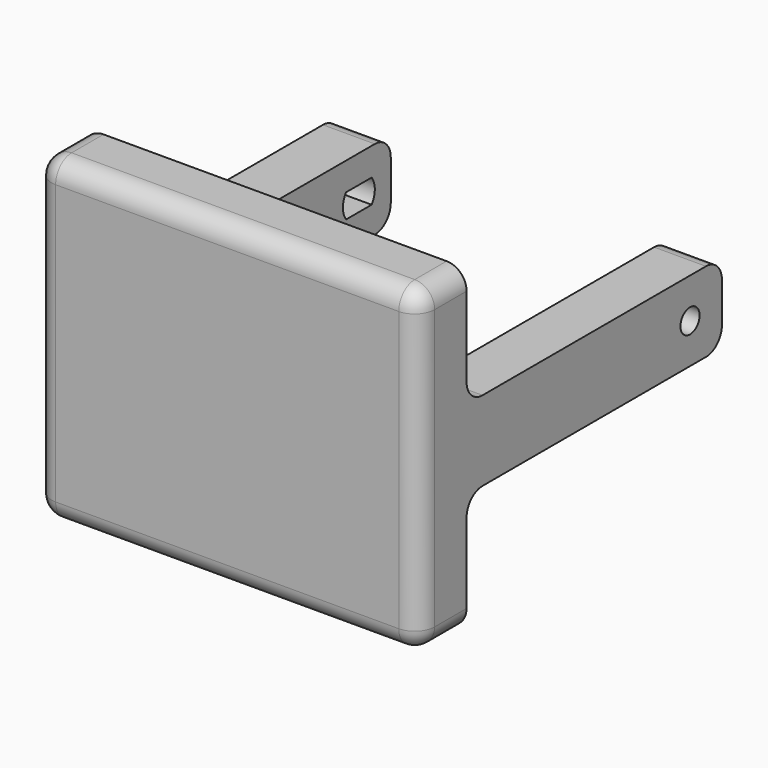
from build123d import *

# Parameters (mm, degrees)
F0_W     = 6.5
F0_H     = 40
F1_DEPTH = 10
F4_DEPTH = 6.5
F2_R     = 1.5
F5_DEPTH = 6.5
F7_DEPTH = 15
F8_DEPTH = 15
F9_R     = 2.5


# Not quite as in the source:
# - a feature names something its author has since deleted; it is built from what else it names


with BuildPart() as f1:
    # F0 (on Top) → F1 (new body)
    with BuildSketch(Plane.XY):
        with Locations((-20.75, 20)):
            Rectangle(F0_W, F0_H)
        with Locations((20.75, 20)):
            Rectangle(F0_W, F0_H)
        Polygon((-17.5, 0), (-24, 0), (-24, -7.5), (24, -7.5), (24, 0), (17.5, 0), align=None)
    extrude(amount=F1_DEPTH)

    # F3 (on face) → F4 (cut, through all)
    with BuildSketch(Plane(origin=(-24, 0, 0), x_dir=(0, -1, 0), z_dir=(-1, 0, 0))):
        with BuildLine():
            ThreePointArc((-33, 3.5), (-32.6282917549, 4.209430585), (-32.5, 5))
            ThreePointArc((-32.5, 5), (-32.6282917549, 5.790569415), (-33, 6.5))
            Line((-33, 6.5), (-37, 6.5))
            ThreePointArc((-37, 6.5), (-37.5, 5), (-37, 3.5))
            Line((-37, 3.5), (-33, 3.5))
        make_face()
    extrude(amount=-F4_DEPTH, mode=Mode.SUBTRACT)

    # F2 (on face) → F5 (cut, through all)
    with BuildSketch(Plane.YZ.offset(24)):
        with Locations((35, 5)):
            Circle(F2_R)
    extrude(amount=-F5_DEPTH, mode=Mode.SUBTRACT)

    # F6 (on face) → F7 (join)
    with BuildSketch(Plane.XY.offset(10)):
        Polygon((-17.5, 0), (-24, 0), (-24, -7.5), (24, -7.5), (24, 0), (17.5, 0), align=None)
    extrude(amount=F7_DEPTH)

    # F0 (on Top) → F8 (join)
    with BuildSketch(Plane.XY):
        Polygon((-17.5, 0), (-24, 0), (-24, -7.5), (24, -7.5), (24, 0), (17.5, 0), align=None)
    extrude(amount=-F8_DEPTH)

    # F9
    f9_edges = [f1.edges().sort_by_distance(p)[0] for p in [
        (-24, -7.5, 5),
        (24, -7.5, 5),
        (-20.75, 40, 10),
        (-20.75, 40, 0),
        (20.75, 40, 10),
        (20.75, 40, 0),
        (0, -7.5, 25),
        (24, -3.75, 25),
        (-24, -3.75, 25),
        (-24, -3.75, -15),
        (24, -3.75, -15),
        (0, -7.5, -15),
        (20.75, 0, 10),
        (20.75, 0, 0),
        (-20.75, 0, 10),
        (-20.75, 0, 0),
    ]]
    fillet(f9_edges, radius=F9_R)


solid = f1.part
